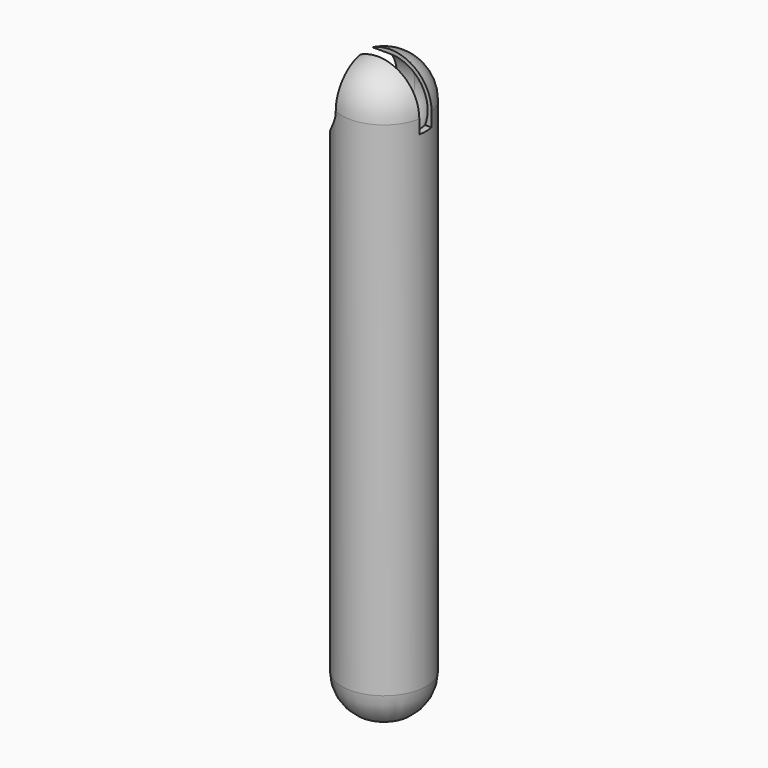
from build123d import *

# Parameters (mm, degrees)
F2_R          = 5
F3_DEPTH      = 5.501
F4_W          = 2
F4_H          = 9
F5_DEPTH      = 12
F5_DEPTH_BACK = 25
F6_R          = 1
F7_DEPTH      = 20


# Not quite as in the source:
# - a fillet or chamfer that OpenCascade refuses, or shapes differently, is made with other operations: its cross-section is extruded or revolved along the edge and cut away or added


with BuildPart() as f1:
    # F0 (on Front) → F1 (revolve)
    with BuildSketch(Plane.XZ):
        with BuildLine():
            Line((0, 5), (0, 5.5))
            ThreePointArc((0, 5.5), (-3.8890872965, 3.8890872965), (-5.5, 0))
            ThreePointArc((-5.5, 0), (-3.8890872965, -3.8890872965), (0, -5.5))
            Line((0, -5.5), (0, -5))
            ThreePointArc((0, -5), (-5, 0), (0, 5))
        make_face()
        with BuildLine():
            Line((0, -70.5), (0, -5.5))
            ThreePointArc((0, -5.5), (-3.8890872965, -3.8890872965), (-5.5, 0))
            Line((-5.5, 0), (-5.5, -70.5))
            Line((-5.5, -70.5), (0, -70.5))
        make_face()
    revolve(axis=Axis((0, 0, -32.5), (0, 0, -1)))

    # F2 (on Right) → F3 (cut, through all)
    with BuildSketch(Plane.YZ):
        Circle(F2_R)
    extrude(amount=-F3_DEPTH, mode=Mode.SUBTRACT)

    # F4 (on Right) → F5 (cut, two sides)
    with BuildSketch(Plane.YZ) as f5_sk:
        with Locations((0, 2.7013579383)):
            Rectangle(F4_W, F4_H)
    extrude(amount=-F5_DEPTH, mode=Mode.SUBTRACT)
    extrude(f5_sk.sketch, amount=F5_DEPTH_BACK, mode=Mode.SUBTRACT)

    # F6 (on face) → F7 (cut)
    with BuildSketch(Plane(origin=(0, 0, -70.5), x_dir=(1, 0, 0), z_dir=(0, 0, -1))):
        Circle(F6_R)
    extrude(amount=-F7_DEPTH, mode=Mode.SUBTRACT)

    # F8: fillet of radius 5 on 1 edges, made by hand

    # F8_s1 → F8_t2 (revolve, cut)
    with BuildSketch(Plane.XZ):
        with BuildLine():
            ThreePointArc((-5.5, -65.5250628145), (-4.2080992435, -68.8791647807), (-1, -70.5))
            Line((-1, -70.5), (-5.5, -70.5))
            Line((-5.5, -70.5), (-5.5, -65.5250628145))
        make_face()
    revolve(axis=Axis((0, 0, -70.5), (0, 0, -1)), mode=Mode.SUBTRACT)


solid = f1.part
